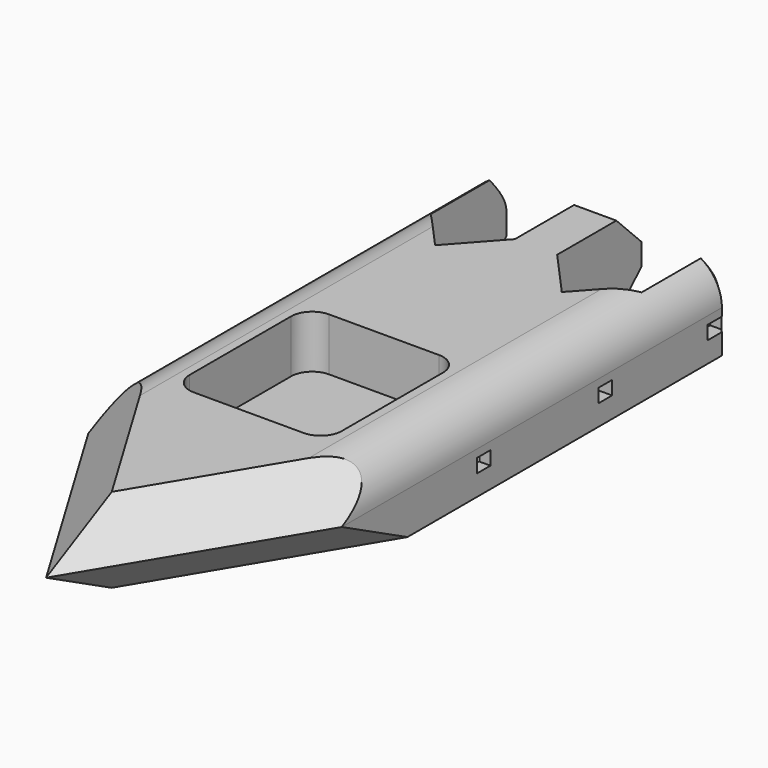
from build123d import *
from build123d import SkipClean  # not in build123d's __all__

# Parameters (mm, degrees)
F0_W        = 2.5
F0_H        = 10
F0_R        = 2.5
F0_W_2      = 3.4
F0_H_2      = 5
F1_DEPTH    = 20
F2_DEPTH    = 7.5
F3_DEPTH    = 6.5
F4_R        = 5
F5_SIZE     = 10
F6_SIZE     = 9.99999
F7_T1_DEPTH = 150.5634936838
F8_SIZE     = 7.5
F9_DEPTH    = 20
F10_START   = 4.9
F10_DEPTH   = 3.24


# Not quite as in the source:
# - a fillet or chamfer that OpenCascade refuses, or shapes differently, is made with other operations: its cross-section is extruded or revolved along the edge and cut away or added
# - a fillet or chamfer is up to 0.001 mm smaller than in the source, because OpenCascade refuses the exact size


with BuildPart() as f1:
    # F0 (on Top) → F1 (new body)
    with BuildSketch(Plane.XY):
        with BuildLine():
            Line((60, 21.2007117721), (50.7183493551, 21.2007117721))
            ThreePointArc((50.7183493551, 21.2007117721), (57.2161836595, 11.5818078095), (59.5, 0.2007117721))
            ThreePointArc((59.5, 0.2007117721), (58.9632243189, -5.4012197743), (57.3724313863, -10.7992882279))
            Line((57.3724313863, -10.7992882279), (60, -10.7992882279))
            Line((60, -10.7992882279), (60, 21.2007117721))
        make_face()
        with BuildLine():
            Line((9.2816506449, 21.2007117721), (0, 21.2007117721))
            Line((0, 21.2007117721), (0, 5.2007117721))
            Line((0, 5.2007117721), (0.9268164798, 5.2007117721))
            ThreePointArc((0.9268164798, 5.2007117721), (3.8504457683, 13.8554110907), (9.2816506449, 21.2007117721))
        make_face()
        with BuildLine():
            Line((2.6275686137, -10.7992882279), (0, -10.7992882279))
            Line((0, -10.7992882279), (0, -14.7992882279))
            Line((0, -14.7992882279), (4.5982284082, -14.7992882279))
            ThreePointArc((4.5982284082, -14.7992882279), (3.5372124485, -12.8365760979), (2.6275686137, -10.7992882279))
        make_face()
        with Locations((46.75, 60.2007117721)):
            Rectangle(F0_W, F0_H)
        with Locations((13.25, 60.2007117721)):
            Rectangle(F0_W, F0_H)
        Polygon((30, -54.7992882279), (30, -104.7992882279), (60, -54.7992882279), (48, -54.7992882279), (43, -54.7992882279), align=None)
        Polygon((12, -54.7992882279), (0, -54.7992882279), (30, -104.7992882279), (30, -54.7992882279), align=None)
        with BuildLine():
            Line((10, 21.2007117721), (9.2816506449, 21.2007117721))
            ThreePointArc((9.2816506449, 21.2007117721), (3.8504457683, 13.8554110907), (0.9268164798, 5.2007117721))
            ThreePointArc((0.9268164798, 5.2007117721), (0.6652618804, -2.9174831312), (2.6275686137, -10.7992882279))
            Line((2.6275686137, -10.7992882279), (10, -10.7992882279))
            Line((10, -10.7992882279), (10, -14.7992882279))
            Line((10, -14.7992882279), (4.5982284082, -14.7992882279))
            ThreePointArc((4.5982284082, -14.7992882279), (7.8990722833, -19.3389656577), (12, -23.1712800129))
            Line((12, -23.1712800129), (12, -4.7992882279))
            Line((12, -4.7992882279), (48, -4.7992882279))
            Line((48, -4.7992882279), (48, -23.1712800129))
            ThreePointArc((48, -23.1712800129), (52.1009277167, -19.3389656577), (55.4017715918, -14.7992882279))
            Line((55.4017715918, -14.7992882279), (50, -14.7992882279))
            Line((50, -14.7992882279), (50, -10.7992882279))
            Line((50, -10.7992882279), (57.3724313863, -10.7992882279))
            ThreePointArc((57.3724313863, -10.7992882279), (58.9632243189, -5.4012197743), (59.5, 0.2007117721))
            ThreePointArc((59.5, 0.2007117721), (57.2161836595, 11.5818078095), (50.7183493551, 21.2007117721))
            Line((50.7183493551, 21.2007117721), (50, 21.2007117721))
            Line((50, 21.2007117721), (50, 21.8859602143))
            ThreePointArc((50, 21.8859602143), (30, 29.7007117721), (10, 21.8859602143))
            Line((10, 21.8859602143), (10, 21.2007117721))
        make_face()
        with Locations((30, 0.2007117721)):
            Circle(F0_R, mode=Mode.SUBTRACT)
        with Locations((30, 0.2007117721)):
            Circle(F0_R)
        Polygon((12, 65.2007117721), (5, 65.2007117721), (5, 40.2007117721), (25, 40.2007117721), (25, 65.2007117721), (14.5, 65.2007117721), (14.5, 55.2007117721), (12, 55.2007117721), align=None)
        Polygon((45.5, 65.2007117721), (35, 65.2007117721), (35, 40.2007117721), (55, 40.2007117721), (55, 65.2007117721), (48, 65.2007117721), (48, 55.2007117721), (45.5, 55.2007117721), align=None)
        Polygon((12, -44.7992882279), (12, -54.7992882279), (30, -54.7992882279), (43, -54.7992882279), (48, -54.7992882279), (48, -44.7992882279), align=None)
        with BuildLine():
            Line((10, 25.2007117721), (0, 25.2007117721))
            Line((0, 25.2007117721), (0, 21.2007117721))
            Line((0, 21.2007117721), (9.2816506449, 21.2007117721))
            ThreePointArc((9.2816506449, 21.2007117721), (9.6379425178, 21.5463580517), (10, 21.8859602143))
            Line((10, 21.8859602143), (10, 25.2007117721))
        make_face()
        with BuildLine():
            Line((4.5982284082, -14.7992882279), (0, -14.7992882279))
            Line((0, -14.7992882279), (0, -49.7992882279))
            Line((0, -49.7992882279), (0, -54.7992882279))
            Line((0, -54.7992882279), (12, -54.7992882279))
            Line((12, -54.7992882279), (12, -44.7992882279))
            Line((12, -44.7992882279), (12, -23.1712800129))
            ThreePointArc((12, -23.1712800129), (7.8990722833, -19.3389656577), (4.5982284082, -14.7992882279))
        make_face()
        with BuildLine():
            Line((10, -10.7992882279), (2.6275686137, -10.7992882279))
            ThreePointArc((2.6275686137, -10.7992882279), (3.5372124485, -12.8365760979), (4.5982284082, -14.7992882279))
            Line((4.5982284082, -14.7992882279), (10, -14.7992882279))
            Line((10, -14.7992882279), (10, -10.7992882279))
        make_face()
        with BuildLine():
            Line((0.9268164798, 5.2007117721), (0, 5.2007117721))
            Line((0, 5.2007117721), (0, -10.7992882279))
            Line((0, -10.7992882279), (2.6275686137, -10.7992882279))
            ThreePointArc((2.6275686137, -10.7992882279), (0.6652618804, -2.9174831312), (0.9268164798, 5.2007117721))
        make_face()
        with BuildLine():
            ThreePointArc((55.4017715918, -14.7992882279), (52.1009277167, -19.3389656577), (48, -23.1712800129))
            Line((48, -23.1712800129), (48, -44.7992882279))
            Line((48, -44.7992882279), (48, -54.7992882279))
            Line((48, -54.7992882279), (60, -54.7992882279))
            Line((60, -54.7992882279), (60, -14.7992882279))
            Line((60, -14.7992882279), (55.4017715918, -14.7992882279))
        make_face()
        with BuildLine():
            Line((5, 65.2007117721), (0, 65.2007117721))
            Line((0, 65.2007117721), (0, 58.455427289))
            Line((0, 58.455427289), (3.4, 58.455427289))
            Line((3.4, 58.455427289), (3.4, 53.455427289))
            Line((3.4, 53.455427289), (0, 53.455427289))
            Line((0, 53.455427289), (0, 25.2007117721))
            Line((0, 25.2007117721), (10, 25.2007117721))
            Line((10, 25.2007117721), (10, 21.8859602143))
            ThreePointArc((10, 21.8859602143), (30, 29.7007117721), (50, 21.8859602143))
            Line((50, 21.8859602143), (50, 25.2007117721))
            Line((50, 25.2007117721), (60, 25.2007117721))
            Line((60, 25.2007117721), (60, 53.455427289))
            Line((60, 53.455427289), (56.6, 53.455427289))
            Line((56.6, 53.455427289), (56.6, 58.455427289))
            Line((56.6, 58.455427289), (60, 58.455427289))
            Line((60, 58.455427289), (60, 65.2007117721))
            Line((60, 65.2007117721), (55, 65.2007117721))
            Line((55, 65.2007117721), (55, 40.2007117721))
            Line((55, 40.2007117721), (45, 29.0628469233))
            Line((45, 29.0628469233), (35, 40.2007117721))
            Line((35, 40.2007117721), (35, 65.2007117721))
            Line((35, 65.2007117721), (30, 65.2007117721))
            Line((30, 65.2007117721), (25, 65.2007117721))
            Line((25, 65.2007117721), (25, 40.2007117721))
            Line((25, 40.2007117721), (15, 29.0628469233))
            Line((15, 29.0628469233), (5, 40.2007117721))
            Line((5, 40.2007117721), (5, 65.2007117721))
        make_face()
        with BuildLine():
            Line((50, 25.2007117721), (50, 21.8859602143))
            ThreePointArc((50, 21.8859602143), (50.3620574822, 21.5463580517), (50.7183493551, 21.2007117721))
            Line((50.7183493551, 21.2007117721), (60, 21.2007117721))
            Line((60, 21.2007117721), (60, 25.2007117721))
            Line((60, 25.2007117721), (50, 25.2007117721))
        make_face()
        with BuildLine():
            Line((60, -10.7992882279), (57.3724313863, -10.7992882279))
            ThreePointArc((57.3724313863, -10.7992882279), (56.4627875515, -12.8365760979), (55.4017715918, -14.7992882279))
            Line((55.4017715918, -14.7992882279), (60, -14.7992882279))
            Line((60, -14.7992882279), (60, -10.7992882279))
        make_face()
        with BuildLine():
            ThreePointArc((55.4017715918, -14.7992882279), (56.4627875515, -12.8365760979), (57.3724313863, -10.7992882279))
            Line((57.3724313863, -10.7992882279), (50, -10.7992882279))
            Line((50, -10.7992882279), (50, -14.7992882279))
            Line((50, -14.7992882279), (55.4017715918, -14.7992882279))
        make_face()
        with BuildLine():
            ThreePointArc((10, 21.8859602143), (9.6379425178, 21.5463580517), (9.2816506449, 21.2007117721))
            Line((9.2816506449, 21.2007117721), (10, 21.2007117721))
            Line((10, 21.2007117721), (10, 21.8859602143))
        make_face()
        with BuildLine():
            ThreePointArc((50.7183493551, 21.2007117721), (50.3620574822, 21.5463580517), (50, 21.8859602143))
            Line((50, 21.8859602143), (50, 21.2007117721))
            Line((50, 21.2007117721), (50.7183493551, 21.2007117721))
        make_face()
        with Locations((1.7, 55.955427289)):
            Rectangle(F0_W_2, F0_H_2)
        with Locations((58.3, 55.955427289)):
            Rectangle(F0_W_2, F0_H_2)
    extrude(amount=F1_DEPTH)

    # F0 (on Top) → F2 (join)
    with BuildSketch(Plane.XY):
        with BuildLine():
            Line((12, -4.7992882279), (12, -23.1712800129))
            ThreePointArc((12, -23.1712800129), (30, -29.2992882279), (48, -23.1712800129))
            Line((48, -23.1712800129), (48, -4.7992882279))
            Line((48, -4.7992882279), (12, -4.7992882279))
        make_face()
        with BuildLine():
            ThreePointArc((48, -23.1712800129), (30, -29.2992882279), (12, -23.1712800129))
            Line((12, -23.1712800129), (12, -44.7992882279))
            Line((12, -44.7992882279), (48, -44.7992882279))
            Line((48, -44.7992882279), (48, -23.1712800129))
        make_face()
    extrude(amount=F2_DEPTH)

    # F0 (on Top) → F3 (cut)
    with BuildSketch(Plane.XY):
        with BuildLine():
            Line((12, -4.7992882279), (12, -23.1712800129))
            ThreePointArc((12, -23.1712800129), (30, -29.2992882279), (48, -23.1712800129))
            Line((48, -23.1712800129), (48, -4.7992882279))
            Line((48, -4.7992882279), (12, -4.7992882279))
        make_face()
        with BuildLine():
            Line((10, 21.2007117721), (9.2816506449, 21.2007117721))
            ThreePointArc((9.2816506449, 21.2007117721), (3.8504457683, 13.8554110907), (0.9268164798, 5.2007117721))
            ThreePointArc((0.9268164798, 5.2007117721), (0.6652618804, -2.9174831312), (2.6275686137, -10.7992882279))
            Line((2.6275686137, -10.7992882279), (10, -10.7992882279))
            Line((10, -10.7992882279), (10, -14.7992882279))
            Line((10, -14.7992882279), (4.5982284082, -14.7992882279))
            ThreePointArc((4.5982284082, -14.7992882279), (7.8990722833, -19.3389656577), (12, -23.1712800129))
            Line((12, -23.1712800129), (12, -4.7992882279))
            Line((12, -4.7992882279), (48, -4.7992882279))
            Line((48, -4.7992882279), (48, -23.1712800129))
            ThreePointArc((48, -23.1712800129), (52.1009277167, -19.3389656577), (55.4017715918, -14.7992882279))
            Line((55.4017715918, -14.7992882279), (50, -14.7992882279))
            Line((50, -14.7992882279), (50, -10.7992882279))
            Line((50, -10.7992882279), (57.3724313863, -10.7992882279))
            ThreePointArc((57.3724313863, -10.7992882279), (58.9632243189, -5.4012197743), (59.5, 0.2007117721))
            ThreePointArc((59.5, 0.2007117721), (57.2161836595, 11.5818078095), (50.7183493551, 21.2007117721))
            Line((50.7183493551, 21.2007117721), (50, 21.2007117721))
            Line((50, 21.2007117721), (50, 21.8859602143))
            ThreePointArc((50, 21.8859602143), (30, 29.7007117721), (10, 21.8859602143))
            Line((10, 21.8859602143), (10, 21.2007117721))
        make_face()
        with Locations((30, 0.2007117721)):
            Circle(F0_R, mode=Mode.SUBTRACT)
        with BuildLine():
            Line((10, -10.7992882279), (2.6275686137, -10.7992882279))
            ThreePointArc((2.6275686137, -10.7992882279), (3.5372124485, -12.8365760979), (4.5982284082, -14.7992882279))
            Line((4.5982284082, -14.7992882279), (10, -14.7992882279))
            Line((10, -14.7992882279), (10, -10.7992882279))
        make_face()
        with BuildLine():
            ThreePointArc((55.4017715918, -14.7992882279), (56.4627875515, -12.8365760979), (57.3724313863, -10.7992882279))
            Line((57.3724313863, -10.7992882279), (50, -10.7992882279))
            Line((50, -10.7992882279), (50, -14.7992882279))
            Line((50, -14.7992882279), (55.4017715918, -14.7992882279))
        make_face()
        with BuildLine():
            ThreePointArc((10, 21.8859602143), (9.6379425178, 21.5463580517), (9.2816506449, 21.2007117721))
            Line((9.2816506449, 21.2007117721), (10, 21.2007117721))
            Line((10, 21.2007117721), (10, 21.8859602143))
        make_face()
        with BuildLine():
            ThreePointArc((50.7183493551, 21.2007117721), (50.3620574822, 21.5463580517), (50, 21.8859602143))
            Line((50, 21.8859602143), (50, 21.2007117721))
            Line((50, 21.2007117721), (50.7183493551, 21.2007117721))
        make_face()
    extrude(amount=F3_DEPTH, mode=Mode.SUBTRACT)

    # F4
    f4_edges = [f1.edges().sort_by_distance(p)[0] for p in [
        (48, -4.799288, 13.75),
        (12, -4.799288, 13.75),
        (12, -44.799288, 13.75),
        (48, -44.799288, 13.75),
    ]]
    fillet(f4_edges, radius=F4_R)

    # F5
    f5_edges = [f1.edges().sort_by_distance(p)[0] for p in [
        (15, -79.799288, 20),
        (45, -79.799288, 20),
    ]]
    chamfer(f5_edges, length=F5_SIZE)

    # F6 (size 10 in the source; OpenCascade refuses exactly that, so slightly less here)
    f6_edges = [f1.edges().sort_by_distance(p)[0] for p in [
        (45, -79.799288, 0),
        (15, -79.799288, 0),
    ]]
    chamfer(f6_edges, length=F6_SIZE)

    # F7: fillet of radius 10 on 2 edges, made by hand

    # F7_s2 → F7_t1 (cut)
    with BuildSketch(Plane.XZ.offset(-90.2007117721)):
        with BuildLine():
            ThreePointArc((50, 20), (57.0710678119, 17.0710678119), (60, 10))
            Line((60, 10), (60, 20))
            Line((60, 20), (50, 20))
        make_face()
        with BuildLine():
            ThreePointArc((0, 10), (2.9289321881, 17.0710678119), (10, 20))
            Line((10, 20), (0, 20))
            Line((0, 20), (0, 10))
        make_face()
    extrude(amount=F7_T1_DEPTH, mode=Mode.SUBTRACT)

    # F8
    f8_edges = [f1.edges().sort_by_distance(p)[0] for p in [
        (30, 65.200712, 20),
        (30, 65.200712, 0),
    ]]
    chamfer(f8_edges, length=F8_SIZE)

    # F0 (on Top) → F9 (cut)
    with BuildSketch(Plane.XY):
        Polygon((12, 65.2007117721), (5, 65.2007117721), (5, 40.2007117721), (25, 40.2007117721), (25, 65.2007117721), (14.5, 65.2007117721), (14.5, 55.2007117721), (12, 55.2007117721), align=None)
        with Locations((13.25, 70.2007117721)):
            Rectangle(F0_W, F0_H)
        with Locations((13.25, 60.2007117721)):
            Rectangle(F0_W, F0_H)
        Polygon((45.5, 65.2007117721), (35, 65.2007117721), (35, 40.2007117721), (55, 40.2007117721), (55, 65.2007117721), (48, 65.2007117721), (48, 55.2007117721), (45.5, 55.2007117721), align=None)
        with Locations((46.75, 60.2007117721)):
            Rectangle(F0_W, F0_H)
        with Locations((46.75, 70.2007117721)):
            Rectangle(F0_W, F0_H)
    with SkipClean():  # cleaning this boolean's faces spoils the solid; the shape is the same uncleaned
        extrude(amount=F9_DEPTH, mode=Mode.SUBTRACT)

    # F0 (on Top) → F10 (cut)
    with BuildSketch(Plane.XY.offset(F10_START)):
        with BuildLine():
            Line((10, 25.2007117721), (0, 25.2007117721))
            Line((0, 25.2007117721), (0, 21.2007117721))
            Line((0, 21.2007117721), (9.2816506449, 21.2007117721))
            ThreePointArc((9.2816506449, 21.2007117721), (9.6379425178, 21.5463580517), (10, 21.8859602143))
            Line((10, 21.8859602143), (10, 25.2007117721))
        make_face()
        with BuildLine():
            Line((50, 25.2007117721), (50, 21.8859602143))
            ThreePointArc((50, 21.8859602143), (50.3620574822, 21.5463580517), (50.7183493551, 21.2007117721))
            Line((50.7183493551, 21.2007117721), (60, 21.2007117721))
            Line((60, 21.2007117721), (60, 25.2007117721))
            Line((60, 25.2007117721), (50, 25.2007117721))
        make_face()
        with BuildLine():
            Line((10, -10.7992882279), (2.6275686137, -10.7992882279))
            ThreePointArc((2.6275686137, -10.7992882279), (3.5372124485, -12.8365760979), (4.5982284082, -14.7992882279))
            Line((4.5982284082, -14.7992882279), (10, -14.7992882279))
            Line((10, -14.7992882279), (10, -10.7992882279))
        make_face()
        with BuildLine():
            Line((2.6275686137, -10.7992882279), (0, -10.7992882279))
            Line((0, -10.7992882279), (0, -14.7992882279))
            Line((0, -14.7992882279), (4.5982284082, -14.7992882279))
            ThreePointArc((4.5982284082, -14.7992882279), (3.5372124485, -12.8365760979), (2.6275686137, -10.7992882279))
        make_face()
        with BuildLine():
            ThreePointArc((55.4017715918, -14.7992882279), (56.4627875515, -12.8365760979), (57.3724313863, -10.7992882279))
            Line((57.3724313863, -10.7992882279), (50, -10.7992882279))
            Line((50, -10.7992882279), (50, -14.7992882279))
            Line((50, -14.7992882279), (55.4017715918, -14.7992882279))
        make_face()
        with BuildLine():
            Line((60, -10.7992882279), (57.3724313863, -10.7992882279))
            ThreePointArc((57.3724313863, -10.7992882279), (56.4627875515, -12.8365760979), (55.4017715918, -14.7992882279))
            Line((55.4017715918, -14.7992882279), (60, -14.7992882279))
            Line((60, -14.7992882279), (60, -10.7992882279))
        make_face()
        with Locations((58.3, 55.955427289)):
            Rectangle(F0_W_2, F0_H_2)
        with Locations((1.7, 55.955427289)):
            Rectangle(F0_W_2, F0_H_2)
    with SkipClean():  # cleaning this boolean's faces spoils the solid; the shape is the same uncleaned
        extrude(amount=F10_DEPTH, mode=Mode.SUBTRACT)


solid = f1.part
